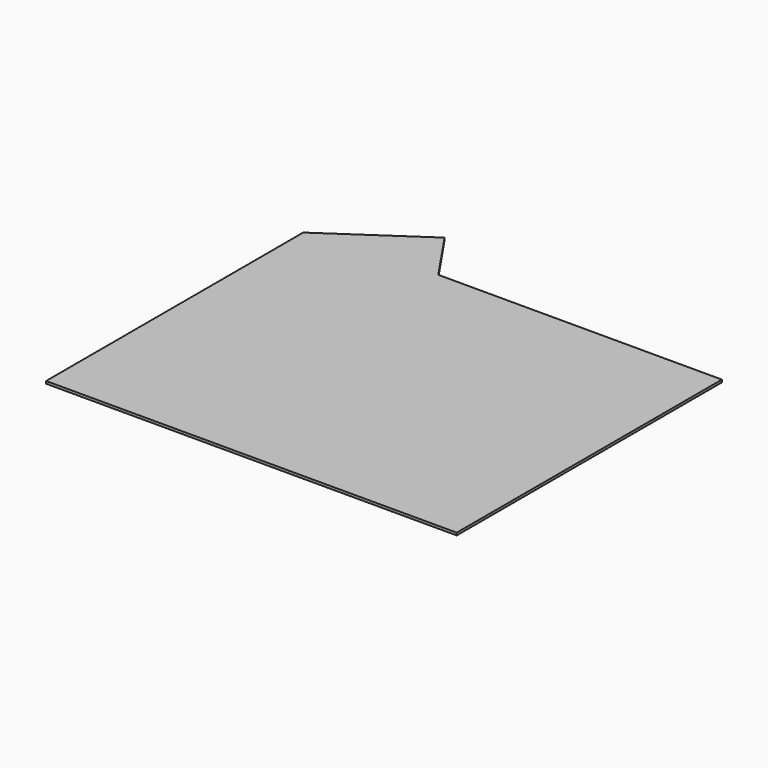
from build123d import *

# Parameters (mm, degrees)
F0_W     = 4216.4
F0_H     = 3403.6
F1_DEPTH = 25.4
F3_DEPTH = 25.4
F5_DEPTH = 25.4


with BuildPart() as f1:
    # F0 (on Top) → F1 (new body)
    with BuildSketch(Plane.XY):
        Rectangle(F0_W, F0_H)
    extrude(amount=F1_DEPTH)

    # F2 (on face) → F3 (join)
    with BuildSketch(Plane.XY.offset(25.4)):
        Polygon((-1168.1525067788, 2237.4002953904), (-1955.8, 1701.8), (-803.9443059133, 1701.8), align=None)
    extrude(amount=-F3_DEPTH)

    # F4 (on face) → F5 (cut)
    with BuildSketch(Plane.XY.offset(25.4)):
        Polygon((-2108.2, 1598.1680001262), (-1955.8, 1701.8), (-2108.2, 1701.8), align=None)
    extrude(amount=-F5_DEPTH, mode=Mode.SUBTRACT)


solid = f1.part
